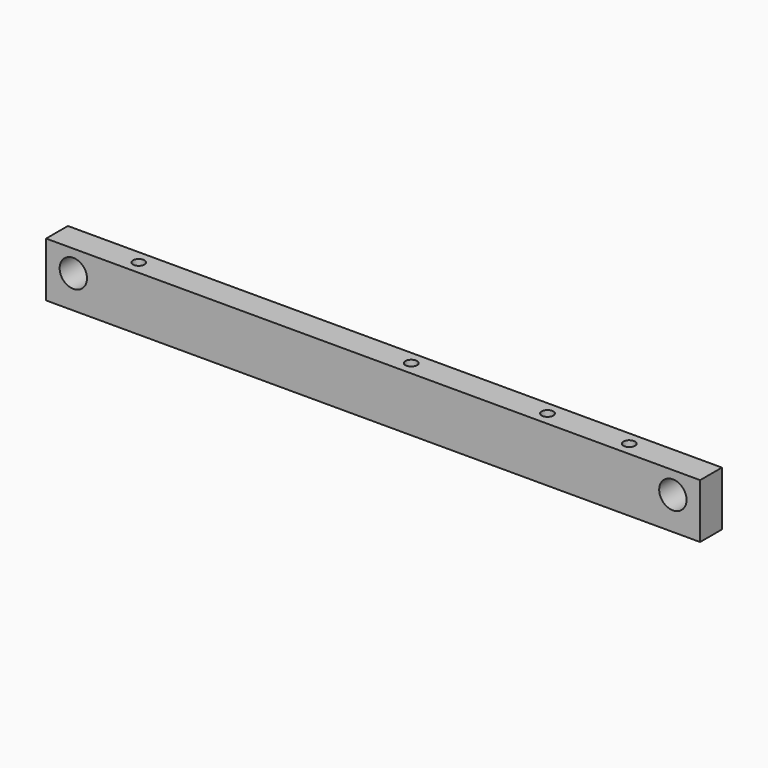
from build123d import *

# Parameters (mm, degrees)
F0_W     = 152.4
F0_H     = 12.7
F0_R     = 3.1877
F1_DEPTH = 6.35
F3_D     = 2.7051
F4_D     = 2.7051
F5_D     = 2.7051


with BuildPart() as f1:
    # F0 (on Front) → F1 (new body)
    with BuildSketch(Plane.XZ):
        Rectangle(F0_W, F0_H)
        with Locations((-69.85, 1.27)):
            Circle(F0_R, mode=Mode.SUBTRACT)
        with Locations((69.85, 1.27)):
            Circle(F0_R, mode=Mode.SUBTRACT)
    extrude(amount=F1_DEPTH)

    # F3 (through all)
    with Locations(Plane(origin=(0, 0, -6.35), x_dir=(1, 0, 0), z_dir=(0, 0, -1))):
        with Locations((-57.15, 3.175), (57.15, 3.175)):
            Hole(F3_D / 2)

    # F4 (through all)
    with Locations(Plane(origin=(0, 0, -6.35), x_dir=(1, 0, 0), z_dir=(0, 0, -1))):
        with Locations((6.35, 3.175)):
            Hole(F4_D / 2)

    # F5 (through all)
    with Locations(Plane(origin=(0, 0, -6.35), x_dir=(1, 0, 0), z_dir=(0, 0, -1))):
        with Locations((38.1, 3.175)):
            Hole(F5_D / 2)


solid = f1.part
